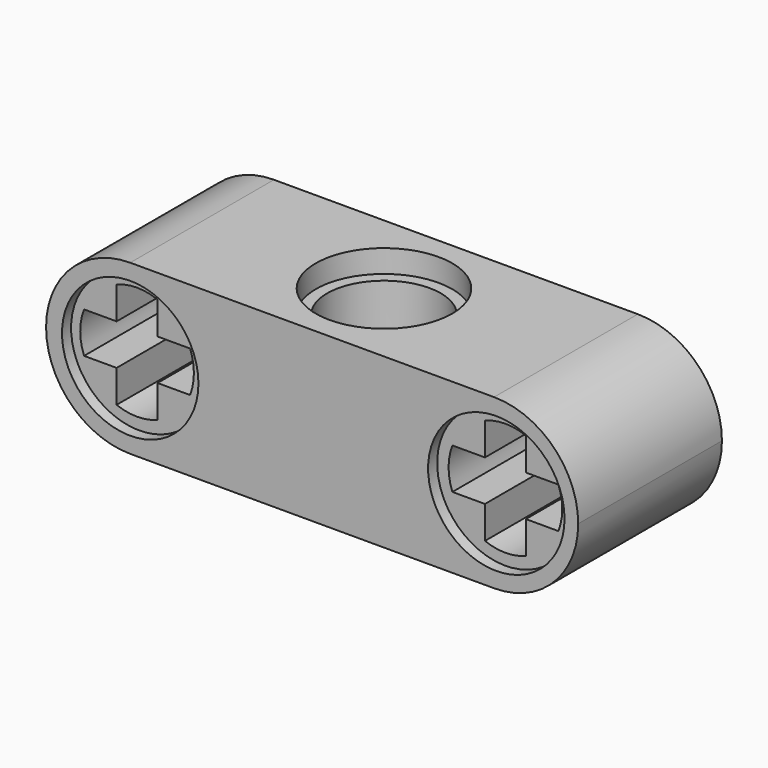
from build123d import *

# Parameters (mm, degrees)
F0_W      = 23.4
F0_H      = 7.4
F1_DEPTH  = 3.95
F2_R      = 3.69999
F3_R      = 2.499
F4_DEPTH  = 25
F3_R_2    = 3
F5_DEPTH  = 1
F6_R      = 3
F6_R_2    = 2.499
F7_DEPTH  = 1
F8_R      = 3
F9_DEPTH  = 0.5
F10_R     = 3
F11_DEPTH = 0.5


# Not quite as in the source:
# - a fillet or chamfer is up to 0.001 mm smaller than in the source, because OpenCascade refuses the exact size


with BuildPart() as f1:
    # F0 (on Front) → F1 (new body, symmetric)
    with BuildSketch(Plane.XZ):
        Rectangle(F0_W, F0_H)
        with BuildLine():
            ThreePointArc((-7.199, -2.3313088598), (-8.099, -2.499), (-8.999, -2.3313088598))
            Line((-8.999, -2.3313088598), (-8.999, -0.9))
            Line((-8.999, -0.9), (-10.4303088598, -0.9))
            ThreePointArc((-10.4303088598, -0.9), (-10.598, 0), (-10.4303088598, 0.9))
            Line((-10.4303088598, 0.9), (-8.999, 0.9))
            Line((-8.999, 0.9), (-8.999, 2.3313088598))
            ThreePointArc((-8.999, 2.3313088598), (-8.099, 2.499), (-7.199, 2.3313088598))
            Line((-7.199, 2.3313088598), (-7.199, 0.9))
            Line((-7.199, 0.9), (-5.7676911402, 0.9))
            ThreePointArc((-5.7676911402, 0.9), (-5.6, 0), (-5.7676911402, -0.9))
            Line((-5.7676911402, -0.9), (-7.199, -0.9))
            Line((-7.199, -0.9), (-7.199, -2.3313088598))
        make_face(mode=Mode.SUBTRACT)
        with BuildLine():
            Line((7.199, 0.9), (7.199, 2.3313088598))
            ThreePointArc((7.199, 2.3313088598), (8.099, 2.499), (8.999, 2.3313088598))
            Line((8.999, 2.3313088598), (8.999, 0.9))
            Line((8.999, 0.9), (10.4303088598, 0.9))
            ThreePointArc((10.4303088598, 0.9), (10.598, 0), (10.4303088598, -0.9))
            Line((10.4303088598, -0.9), (8.999, -0.9))
            Line((8.999, -0.9), (8.999, -2.3313088598))
            ThreePointArc((8.999, -2.3313088598), (8.099, -2.499), (7.199, -2.3313088598))
            Line((7.199, -2.3313088598), (7.199, -0.9))
            Line((7.199, -0.9), (5.7676911402, -0.9))
            ThreePointArc((5.7676911402, -0.9), (5.6, 0), (5.7676911402, 0.9))
            Line((5.7676911402, 0.9), (7.199, 0.9))
        make_face(mode=Mode.SUBTRACT)
    extrude(amount=F1_DEPTH, both=True)

    # F2 (radius 3.7 in the source; OpenCascade refuses exactly that, so slightly less here)
    f2_edges = [f1.edges().sort_by_distance(p)[0] for p in [
        (-11.7, 0, -3.7),
        (-11.7, 0, 3.7),
        (11.7, 0, 3.7),
        (11.7, 0, -3.7),
    ]]
    fillet(f2_edges, radius=F2_R)

    # F3 (on face) → F4 (cut)
    with BuildSketch(Plane.XY.offset(3.7)):
        Circle(F3_R)
    extrude(amount=-F4_DEPTH, mode=Mode.SUBTRACT)

    # F3 (on face) → F5 (cut)
    with BuildSketch(Plane.XY.offset(3.7)):
        Circle(F3_R_2)
        Circle(F3_R, mode=Mode.SUBTRACT)
    extrude(amount=-F5_DEPTH, mode=Mode.SUBTRACT)

    # F6 (on face) → F7 (cut)
    with BuildSketch(Plane(origin=(0, 0, -3.7), x_dir=(1, 0, 0), z_dir=(0, 0, -1))):
        Circle(F6_R)
        Circle(F6_R_2, mode=Mode.SUBTRACT)
    extrude(amount=-F7_DEPTH, mode=Mode.SUBTRACT)

    # F8 (on face) → F9 (cut)
    with BuildSketch(Plane.XZ.offset(3.95)):
        with Locations((-8, 0)):
            Circle(F8_R)
        with Locations((8.099, 0)):
            Circle(F8_R)
    extrude(amount=-F9_DEPTH, mode=Mode.SUBTRACT)

    # F10 (on face) → F11 (cut)
    with BuildSketch(Plane(origin=(0, 3.95, 0), x_dir=(-1, 0, 0), z_dir=(0, 1, 0))):
        with Locations((-8, 0)):
            Circle(F10_R)
        with Locations((8.099, 0)):
            Circle(F10_R)
    extrude(amount=-F11_DEPTH, mode=Mode.SUBTRACT)


solid = f1.part
